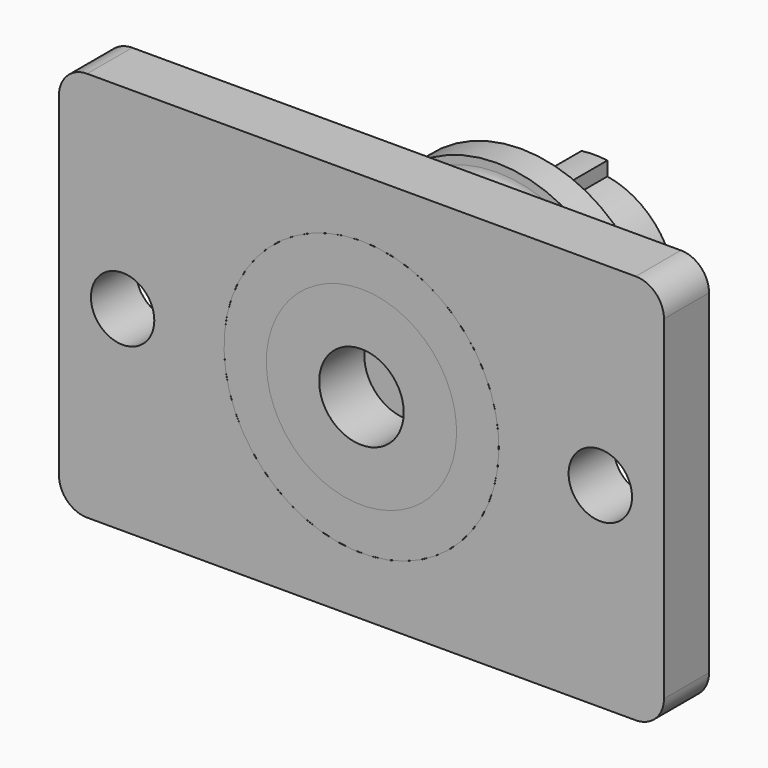
from build123d import *

# Parameters (mm, degrees)
F0_R     = 1.7145
F0_R_2   = 7.4295
F1_DEPTH = 3.048
F0_R_3   = 2.286
F0_R_4   = 2.032
F0_R_5   = 0.635
F2_DEPTH = 12.7
F0_R_6   = 5.969
F3_DEPTH = 3.048
F6_R     = 1.016


# Not quite as in the source:
# - a feature of the source that left no trace in its solid (it failed there, or was rolled back) is left out
# - a feature names something its author has since deleted; it is built from what else it names
# - the program builds the solid bodies; features that only make, move or delete a surface that nothing else refers to are left out


with BuildPart() as f1:
    # F0 (on Front) → F1 (new body)
    with BuildSketch(Plane.XZ):
        with BuildLine():
            ThreePointArc((16.3576, 9.0424), (15.9112307345, 10.1200307345), (14.8336, 10.5664))
            Line((14.8336, 10.5664), (-14.8336, 10.5664))
            ThreePointArc((-14.8336, 10.5664), (-15.9112307345, 10.1200307345), (-16.3576, 9.0424))
            Line((-16.3576, 9.0424), (-16.3576, -9.0424))
            ThreePointArc((-16.3576, -9.0424), (-15.9112307345, -10.1200307345), (-14.8336, -10.5664))
            Line((-14.8336, -10.5664), (14.8336, -10.5664))
            ThreePointArc((14.8336, -10.5664), (15.9112307345, -10.1200307345), (16.3576, -9.0424))
            Line((16.3576, -9.0424), (16.3576, 9.0424))
        make_face()
        with Locations((-12.9159, 0)):
            Circle(F0_R, mode=Mode.SUBTRACT)
        Circle(F0_R_2, mode=Mode.SUBTRACT)
        with Locations((12.9159, 0)):
            Circle(F0_R, mode=Mode.SUBTRACT)
    extrude(amount=F1_DEPTH)


with BuildPart() as f2:
    # F0 (on Front) → F2 (new body)
    with BuildSketch(Plane.XZ):
        with BuildLine():
            ThreePointArc((4.3254641369, -0.6985), (4.3674685669, -0.3503720408), (4.3815, 0))
            ThreePointArc((4.3815, 0), (4.3674685669, 0.3503720408), (4.3254641369, 0.6985))
            ThreePointArc((4.3254641369, 0.6985), (3.0981883618, 3.0981883618), (0.6985, 4.3254641369))
            ThreePointArc((0.6985, 4.3254641369), (0, 4.3815), (-0.6985, 4.3254641369))
            ThreePointArc((-0.6985, 4.3254641369), (-3.0981883618, 3.0981883618), (-4.3254641369, 0.6985))
            ThreePointArc((-4.3254641369, 0.6985), (-4.3815, 0), (-4.3254641369, -0.6985))
            ThreePointArc((-4.3254641369, -0.6985), (-3.139825836, -3.0559836338), (-0.8152878707, -4.3049794352))
            ThreePointArc((-0.8152878707, -4.3049794352), (0, -4.3815), (0.8152878707, -4.3049794352))
            ThreePointArc((0.8152878707, -4.3049794352), (3.139825836, -3.0559836338), (4.3254641369, -0.6985))
        make_face()
        Circle(F0_R_3, mode=Mode.SUBTRACT)
        Circle(F0_R_3)
        Circle(F0_R_4, mode=Mode.SUBTRACT)
        Circle(F0_R_4)
        Circle(F0_R_5, mode=Mode.SUBTRACT)
        with BuildLine():
            Line((0.8152878707, -5.0700591005), (0.8152878707, -4.3049794352))
            ThreePointArc((0.8152878707, -4.3049794352), (0, -4.3815), (-0.8152878707, -4.3049794352))
            Line((-0.8152878707, -4.3049794352), (-0.8152878707, -5.0700591005))
            ThreePointArc((-0.8152878707, -5.0700591005), (0, -5.1351916804), (0.8152878707, -5.0700591005))
        make_face()
        with BuildLine():
            ThreePointArc((4.3254641369, 0.6985), (4.3674685669, 0.3503720408), (4.3815, 0))
            ThreePointArc((4.3815, 0), (4.3674685669, -0.3503720408), (4.3254641369, -0.6985))
            Line((4.3254641369, -0.6985), (5.0874641369, -0.6985))
            ThreePointArc((5.0874641369, -0.6985), (5.1351916804, 0), (5.0874641369, 0.6985))
            Line((5.0874641369, 0.6985), (4.3254641369, 0.6985))
        make_face()
        with BuildLine():
            ThreePointArc((-0.6985, 4.3254641369), (0, 4.3815), (0.6985, 4.3254641369))
            Line((0.6985, 4.3254641369), (0.6985, 5.0874641369))
            ThreePointArc((0.6985, 5.0874641369), (0, 5.1351916804), (-0.6985, 5.0874641369))
            Line((-0.6985, 5.0874641369), (-0.6985, 4.3254641369))
        make_face()
        with BuildLine():
            ThreePointArc((-4.3254641369, -0.6985), (-4.3815, 0), (-4.3254641369, 0.6985))
            Line((-4.3254641369, 0.6985), (-5.0874641369, 0.6985))
            ThreePointArc((-5.0874641369, 0.6985), (-5.1351916804, 0), (-5.0874641369, -0.6985))
            Line((-5.0874641369, -0.6985), (-4.3254641369, -0.6985))
        make_face()
    extrude(amount=-F2_DEPTH)


with BuildPart() as f3:
    # F0 (on Front) → F3 (new body)
    with BuildSketch(Plane.XZ):
        Circle(F0_R_6)
        with BuildLine():
            ThreePointArc((0.6985, 5.0874641369), (3.6311288599, 3.6311288599), (5.0874641369, 0.6985))
            ThreePointArc((5.0874641369, 0.6985), (5.1351916804, 0), (5.0874641369, -0.6985))
            ThreePointArc((5.0874641369, -0.6985), (3.6726356419, -3.5891421031), (0.8152878707, -5.0700591005))
            ThreePointArc((0.8152878707, -5.0700591005), (0, -5.1351916804), (-0.8152878707, -5.0700591005))
            ThreePointArc((-0.8152878707, -5.0700591005), (-3.6726356419, -3.5891421031), (-5.0874641369, -0.6985))
            ThreePointArc((-5.0874641369, -0.6985), (-5.1351916804, 0), (-5.0874641369, 0.6985))
            ThreePointArc((-5.0874641369, 0.6985), (-3.6311288599, 3.6311288599), (-0.6985, 5.0874641369))
            ThreePointArc((-0.6985, 5.0874641369), (0, 5.1351916804), (0.6985, 5.0874641369))
        make_face(mode=Mode.SUBTRACT)
        with BuildLine():
            ThreePointArc((4.3254641369, -0.6985), (4.3674685669, -0.3503720408), (4.3815, 0))
            ThreePointArc((4.3815, 0), (4.3674685669, 0.3503720408), (4.3254641369, 0.6985))
            ThreePointArc((4.3254641369, 0.6985), (3.0981883618, 3.0981883618), (0.6985, 4.3254641369))
            ThreePointArc((0.6985, 4.3254641369), (0, 4.3815), (-0.6985, 4.3254641369))
            ThreePointArc((-0.6985, 4.3254641369), (-3.0981883618, 3.0981883618), (-4.3254641369, 0.6985))
            ThreePointArc((-4.3254641369, 0.6985), (-4.3815, 0), (-4.3254641369, -0.6985))
            ThreePointArc((-4.3254641369, -0.6985), (-3.139825836, -3.0559836338), (-0.8152878707, -4.3049794352))
            ThreePointArc((-0.8152878707, -4.3049794352), (0, -4.3815), (0.8152878707, -4.3049794352))
            ThreePointArc((0.8152878707, -4.3049794352), (3.139825836, -3.0559836338), (4.3254641369, -0.6985))
        make_face()
        Circle(F0_R_3, mode=Mode.SUBTRACT)
        with BuildLine():
            ThreePointArc((0.6985, 4.3254641369), (3.0981883618, 3.0981883618), (4.3254641369, 0.6985))
            Line((4.3254641369, 0.6985), (5.0874641369, 0.6985))
            ThreePointArc((5.0874641369, 0.6985), (3.6311288599, 3.6311288599), (0.6985, 5.0874641369))
            Line((0.6985, 5.0874641369), (0.6985, 4.3254641369))
        make_face()
        with BuildLine():
            ThreePointArc((-4.3254641369, 0.6985), (-3.0981883618, 3.0981883618), (-0.6985, 4.3254641369))
            Line((-0.6985, 4.3254641369), (-0.6985, 5.0874641369))
            ThreePointArc((-0.6985, 5.0874641369), (-3.6311288599, 3.6311288599), (-5.0874641369, 0.6985))
            Line((-5.0874641369, 0.6985), (-4.3254641369, 0.6985))
        make_face()
        with BuildLine():
            Line((5.0874641369, -0.6985), (4.3254641369, -0.6985))
            ThreePointArc((4.3254641369, -0.6985), (3.139825836, -3.0559836338), (0.8152878707, -4.3049794352))
            Line((0.8152878707, -4.3049794352), (0.8152878707, -5.0700591005))
            ThreePointArc((0.8152878707, -5.0700591005), (3.6726356419, -3.5891421031), (5.0874641369, -0.6985))
        make_face()
        with BuildLine():
            Line((-0.8152878707, -5.0700591005), (-0.8152878707, -4.3049794352))
            ThreePointArc((-0.8152878707, -4.3049794352), (-3.139825836, -3.0559836338), (-4.3254641369, -0.6985))
            Line((-4.3254641369, -0.6985), (-5.0874641369, -0.6985))
            ThreePointArc((-5.0874641369, -0.6985), (-3.6726356419, -3.5891421031), (-0.8152878707, -5.0700591005))
        make_face()
        with BuildLine():
            Line((0.8152878707, -5.0700591005), (0.8152878707, -4.3049794352))
            ThreePointArc((0.8152878707, -4.3049794352), (0, -4.3815), (-0.8152878707, -4.3049794352))
            Line((-0.8152878707, -4.3049794352), (-0.8152878707, -5.0700591005))
            ThreePointArc((-0.8152878707, -5.0700591005), (0, -5.1351916804), (0.8152878707, -5.0700591005))
        make_face()
        with BuildLine():
            ThreePointArc((4.3254641369, 0.6985), (4.3674685669, 0.3503720408), (4.3815, 0))
            ThreePointArc((4.3815, 0), (4.3674685669, -0.3503720408), (4.3254641369, -0.6985))
            Line((4.3254641369, -0.6985), (5.0874641369, -0.6985))
            ThreePointArc((5.0874641369, -0.6985), (5.1351916804, 0), (5.0874641369, 0.6985))
            Line((5.0874641369, 0.6985), (4.3254641369, 0.6985))
        make_face()
        with BuildLine():
            ThreePointArc((-4.3254641369, -0.6985), (-4.3815, 0), (-4.3254641369, 0.6985))
            Line((-4.3254641369, 0.6985), (-5.0874641369, 0.6985))
            ThreePointArc((-5.0874641369, 0.6985), (-5.1351916804, 0), (-5.0874641369, -0.6985))
            Line((-5.0874641369, -0.6985), (-4.3254641369, -0.6985))
        make_face()
        with BuildLine():
            ThreePointArc((-0.6985, 4.3254641369), (0, 4.3815), (0.6985, 4.3254641369))
            Line((0.6985, 4.3254641369), (0.6985, 5.0874641369))
            ThreePointArc((0.6985, 5.0874641369), (0, 5.1351916804), (-0.6985, 5.0874641369))
            Line((-0.6985, 5.0874641369), (-0.6985, 4.3254641369))
        make_face()
    extrude(amount=F3_DEPTH)


with BuildPart() as f5:
    # F4 (on Right) → F5 (revolve)
    with BuildSketch(Plane.YZ):
        Polygon((-3.048, 7.4295), (-3.048, 5.1435), (7.747, 5.1435), (7.747, 7.4295), (6.096, 7.4295), (6.096, 5.969), (3.937, 5.969), (3.937, 7.4295), align=None)
    revolve(axis=Axis((0, 9.7803371027, 0), (0, 1, 0)))

    # F6
    f6_edges = [f5.edges().sort_by_distance(p)[0] for p in [
        (0, 6.096, -5.969),
        (0, 3.937, -5.969),
    ]]
    fillet(f6_edges, radius=F6_R)


solid = Compound([f1.part, f2.part, f3.part, f5.part])
